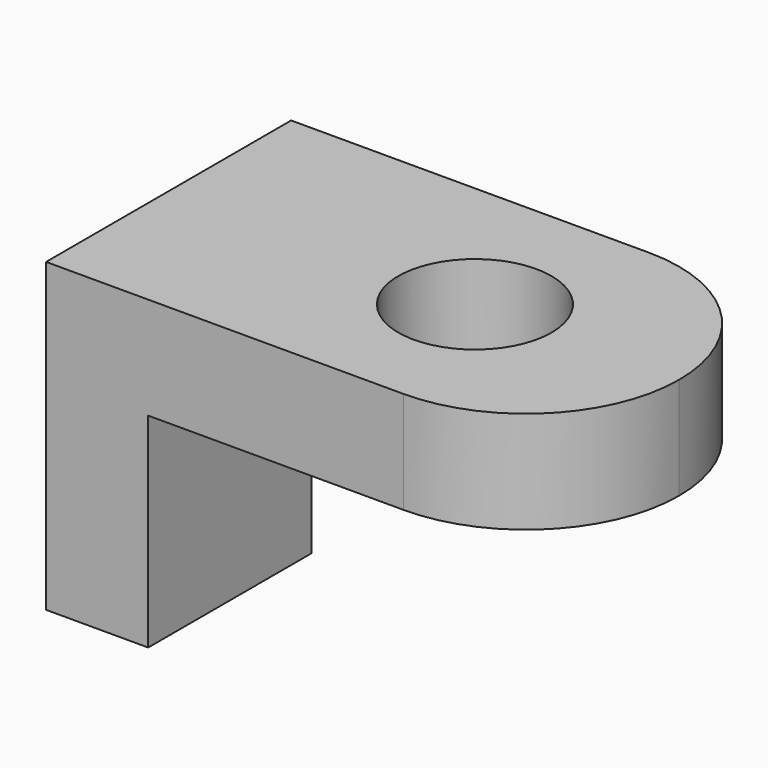
from build123d import *

# Parameters (mm, degrees)
F0_W     = 101.6
F0_H     = 76.2
F1_DEPTH = 25.4
F2_R     = 38.09999
F3_R     = 19.05
F4_DEPTH = 25.401
F5_W     = 25.4
F5_H     = 76.2
F6_DEPTH = 76.2
F7_W     = 25.4
F7_H     = 25.4
F8_DEPTH = 25.4


# Not quite as in the source:
# - a fillet or chamfer is up to 0.001 mm smaller than in the source, because OpenCascade refuses the exact size


with BuildPart() as f1:
    # F0 (on Top) → F1 (new body)
    with BuildSketch(Plane.XY):
        Rectangle(F0_W, F0_H)
    extrude(amount=F1_DEPTH)

    # F2 (radius 38.1 in the source; OpenCascade refuses exactly that, so slightly less here)
    f2_edges = [f1.edges().sort_by_distance(p)[0] for p in [
        (50.8, -38.1, 12.7),
        (50.8, 38.1, 12.7),
    ]]
    fillet(f2_edges, radius=F2_R)

    # F3 (on Top) → F4 (cut, through all)
    with BuildSketch(Plane.XY):
        Circle(F3_R)
    extrude(amount=F4_DEPTH, mode=Mode.SUBTRACT)

    # F5 (on face) → F6 (join)
    with BuildSketch(Plane.XY.offset(25.4)):
        with Locations((-63.5, 0)):
            Rectangle(F5_W, F5_H)
    extrude(amount=-F6_DEPTH)

    # F7 (on face) → F8 (cut)
    with BuildSketch(Plane.YZ.offset(-50.8)):
        with Locations((25.4, -38.1)):
            Rectangle(F7_W, F7_H)
    extrude(amount=-F8_DEPTH, mode=Mode.SUBTRACT)


solid = f1.part
